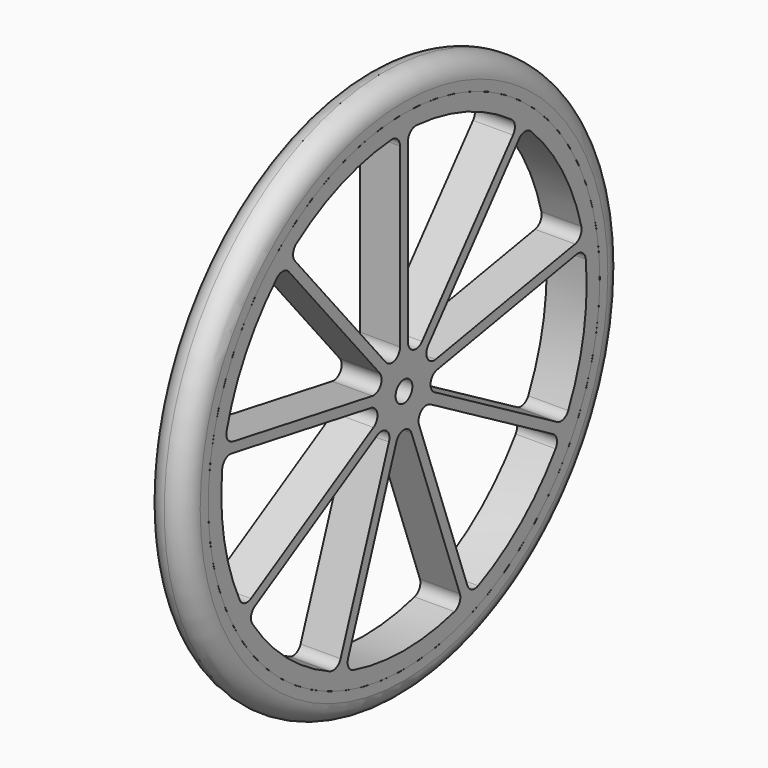
from build123d import *

# Parameters (mm, degrees)
F0_W     = 40
F0_H     = 245
F3_R     = 10.5
F4_DEPTH = 79
F5_R     = 275
F5_R_2   = 245
F6_DEPTH = 40
F7_R     = 19.99999


# Not quite as in the source:
# - a fillet or chamfer is up to 0.001 mm smaller than in the source, because OpenCascade refuses the exact size


with BuildPart() as f1:
    # F0 (on Front) → F1 (revolve)
    with BuildSketch(Plane.XZ):
        with Locations((0, 122.5)):
            Rectangle(F0_W, F0_H)
    revolve(axis=Axis((0, 0, 0), (1, 0, 0)))

    # F3 (on face) → F4 (cut)
    with BuildSketch(Plane.YZ.offset(20)):
        with BuildLine():
            ThreePointArc((15.7661695952, 228.1581450576), (8.205211407, 225.524489914), (5, 218.1875390503))
            Line((5, 218.1875390503), (5, 41.2121612918))
            ThreePointArc((5, 41.2121612918), (11.5797985667, 31.815235084), (22.6604444312, 34.784285195))
            Line((22.6604444312, 34.784285195), (136.418024474, 170.3552898957))
            ThreePointArc((136.418024474, 170.3552898957), (138.6787911947, 178.0359905131), (134.5796420844, 184.9135776417))
            ThreePointArc((134.5796420844, 184.9135776417), (78.1359177886, 214.6766697724), (15.7661695952, 228.1581450576))
        make_face()
        with BuildLine():
            ThreePointArc((-5, 218.1875390503), (-8.205211407, 225.524489914), (-15.7661695952, 228.1581450576))
            ThreePointArc((-15.7661695952, 228.1581450576), (-78.1359177886, 214.6766697724), (-134.5796420844, 184.9135776417))
            ThreePointArc((-134.5796420844, 184.9135776417), (-138.6787911947, 178.0359905131), (-136.418024474, 170.3552898957))
            Line((-136.418024474, 170.3552898957), (-22.6604444312, 34.784285195))
            ThreePointArc((-22.6604444312, 34.784285195), (-11.5797985667, 31.815235084), (-5, 41.2121612918))
            Line((-5, 41.2121612918), (-5, 218.1875390503))
        make_face()
        with BuildLine():
            ThreePointArc((-144.0784689051, 163.9274137989), (-151.2499044005, 167.4875740586), (-158.7348152998, 164.6449807056))
            ThreePointArc((-158.7348152998, 164.6449807056), (-197.8470890484, 114.2270701205), (-221.9541435466, 55.1458921618))
            ThreePointArc((-221.9541435466, 55.1458921618), (-220.6734461533, 47.2424725015), (-214.0045391791, 42.8119073108))
            Line((-214.0045391791, 42.8119073108), (-39.7178150702, 12.0804554711))
            ThreePointArc((-39.7178150702, 12.0804554711), (-29.3210792557, 16.9285330012), (-30.3208888624, 28.3564090981))
            Line((-30.3208888624, 28.3564090981), (-144.0784689051, 163.9274137989))
        make_face()
        with BuildLine():
            ThreePointArc((-215.7410209558, 32.9638297807), (-223.5230861696, 31.0813608841), (-227.4296767846, 24.0926000564))
            ThreePointArc((-227.4296767846, 24.0926000564), (-224.9834085171, -39.6706451333), (-205.4738344978, -100.4251691389))
            ThreePointArc((-205.4738344978, -100.4251691389), (-199.4125431446, -105.6563234351), (-191.4559516068, -104.7636425062))
            Line((-191.4559516068, -104.7636425062), (-38.1907786236, -16.275953627))
            ThreePointArc((-38.1907786236, -16.275953627), (-33.3427010935, -5.8792178125), (-41.4542968469, 2.232377941))
            Line((-41.4542968469, 2.232377941), (-215.7410209558, 32.9638297807))
        make_face()
        with BuildLine():
            ThreePointArc((-186.4559516068, -113.4238965441), (-191.2073317376, -119.8681664789), (-189.7076649026, -127.7329759186))
            ThreePointArc((-189.7076649026, -127.7329759186), (-146.8474907285, -175.0060246391), (-92.8500347002, -209.0061776981))
            ThreePointArc((-92.8500347002, -209.0061776981), (-84.844294975, -209.1173513973), (-79.3229964818, -203.3191196764))
            Line((-79.3229964818, -203.3191196764), (-18.7938524157, -37.0166631359))
            ThreePointArc((-18.7938524157, -37.0166631359), (-21.7629025267, -25.9360172715), (-33.1907786236, -24.9362076648))
            Line((-33.1907786236, -24.9362076648), (-186.4559516068, -113.4238965441))
        make_face()
        with BuildLine():
            ThreePointArc((-69.9260702739, -206.7393211097), (-69.4235417527, -214.7300465601), (-63.2193282468, -219.7908728675))
            ThreePointArc((-63.2193282468, -219.7908728675), (0, -228.454140241), (63.2193282468, -219.7908728675))
            ThreePointArc((63.2193282468, -219.7908728675), (69.4235417527, -214.7300465601), (69.9260702739, -206.7393211097))
            Line((69.9260702739, -206.7393211097), (9.3969262079, -40.4368645692))
            ThreePointArc((9.3969262079, -40.4368645692), (0, -33.8570660024), (-9.3969262079, -40.4368645692))
            Line((-9.3969262079, -40.4368645692), (-69.9260702739, -206.7393211097))
        make_face()
        with BuildLine():
            ThreePointArc((79.3229964818, -203.3191196764), (84.844294975, -209.1173513973), (92.8500347002, -209.0061776981))
            ThreePointArc((92.8500347002, -209.0061776981), (146.8474907285, -175.0060246391), (189.7076649026, -127.7329759186))
            ThreePointArc((189.7076649026, -127.7329759186), (191.2073317376, -119.8681664789), (186.4559516068, -113.4238965441))
            Line((186.4559516068, -113.4238965441), (33.1907786236, -24.9362076648))
            ThreePointArc((33.1907786236, -24.9362076648), (21.7629025267, -25.9360172715), (18.7938524157, -37.0166631359))
            Line((18.7938524157, -37.0166631359), (79.3229964818, -203.3191196764))
        make_face()
        with BuildLine():
            ThreePointArc((191.4559516068, -104.7636425062), (199.4125431446, -105.6563234351), (205.4738344978, -100.4251691389))
            ThreePointArc((205.4738344978, -100.4251691389), (224.9834085171, -39.6706451333), (227.4296767846, 24.0926000564))
            ThreePointArc((227.4296767846, 24.0926000564), (223.5230861696, 31.0813608841), (215.7410209558, 32.9638297807))
            Line((215.7410209558, 32.9638297807), (41.4542968469, 2.232377941))
            ThreePointArc((41.4542968469, 2.232377941), (33.3427010935, -5.8792178125), (38.1907786236, -16.275953627))
            Line((38.1907786236, -16.275953627), (191.4559516068, -104.7636425062))
        make_face()
        with BuildLine():
            ThreePointArc((214.0045391791, 42.8119073108), (220.6734461533, 47.2424725015), (221.9541435466, 55.1458921618))
            ThreePointArc((221.9541435466, 55.1458921618), (197.8470890484, 114.2270701205), (158.7348152998, 164.6449807056))
            ThreePointArc((158.7348152998, 164.6449807056), (151.2499044005, 167.4875740586), (144.0784689051, 163.9274137989))
            Line((144.0784689051, 163.9274137989), (30.3208888624, 28.3564090981))
            ThreePointArc((30.3208888624, 28.3564090981), (29.3210792557, 16.9285330012), (39.7178150702, 12.0804554711))
            Line((39.7178150702, 12.0804554711), (214.0045391791, 42.8119073108))
        make_face()
        Circle(F3_R)
    extrude(amount=-F4_DEPTH, mode=Mode.SUBTRACT)


with BuildPart() as f6:
    # F5 (on face) → F6 (new body)
    with BuildSketch(Plane.YZ.offset(20)):
        Circle(F5_R)
        Circle(F5_R_2, mode=Mode.SUBTRACT)
    extrude(amount=-F6_DEPTH)

    # F7 (radius 20 in the source; OpenCascade refuses exactly that, so slightly less here)
    f7_edges = [f6.edges().sort_by_distance(p)[0] for p in [
        (-20, -275, 0),
        (20, -275, 0),
    ]]
    fillet(f7_edges, radius=F7_R)


solid = Compound([f1.part, f6.part])
